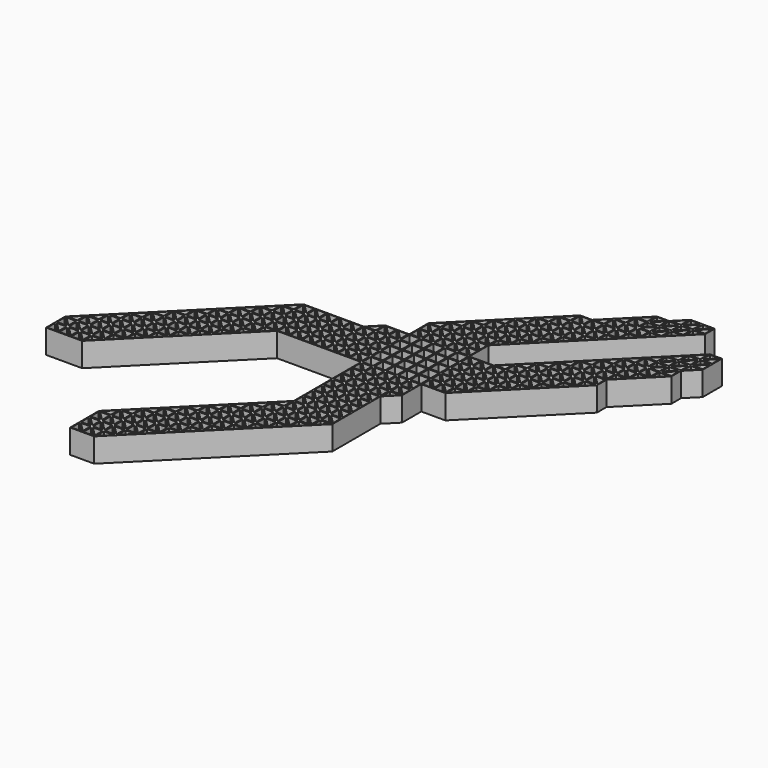
from build123d import *

# Parameters (mm, degrees)
F0_W     = 4.399904
F0_H     = 4.399732
F0_W_2   = 4.399732
F0_H_2   = 4.399903
F0_W_3   = 4.399903
F0_H_3   = 4.399904
F0_H_4   = 4.399731
F1_DEPTH = 5


with BuildPart() as f1:
    # F0 (on Top) → F1 (new body, symmetric)
    with BuildSketch(Plane.XY):
        Polygon((-42.49999, -77.500007), (-42.49999, -92.499952), (-32.500084, -92.499952), (22.500004, -37.500037), (22.500004, -12.500012), (27.500044, -7.500145), (27.500044, 2.499934), (37.500122, 2.499934), (72.500053, 37.500037), (72.500053, 42.499904), (87.499999, 57.500022), (87.499999, 62.500061), (92.500038, 67.499928), (92.500038, 77.500007), (87.499999, 77.500007), (37.49995, 27.499958), (27.500044, 27.499958), (27.500044, 37.500037), (77.500093, 87.499913), (77.500093, 92.499953), (67.500014, 92.499953), (62.499975, 87.499913), (57.500108, 87.499913), (42.49999, 72.499968), (37.500122, 72.499968), (2.500019, 37.499864), (2.500019, 27.499958), (-7.499887, 27.499958), (-12.499926, 22.499919), (-37.499951, 22.499919), (-92.500039, -32.499997), (-92.500039, -42.500076), (-77.500093, -42.500076), (-32.500084, 2.499934), (2.500019, 2.499934), (2.500019, -32.499997), align=None)
        Polygon((-42.200267, -92.199885), (-42.200267, -88.224244), (-38.224454, -92.199885), align=None, mode=Mode.SUBTRACT)
        Polygon((-37.800191, -91.775793), (-41.776003, -87.800153), (-37.800191, -87.800153), align=None, mode=Mode.SUBTRACT)
        Polygon((-37.200055, -92.199885), (-37.200055, -88.224244), (-33.224415, -92.199885), align=None, mode=Mode.SUBTRACT)
        Polygon((-36.77493, -87.800498), (-32.800496, -87.800153), (-32.800496, -91.775104), align=None, mode=Mode.SUBTRACT)
        Polygon((-42.200784, -87.200018), (-42.200784, -83.224377), (-38.224971, -87.200018), align=None, mode=Mode.SUBTRACT)
        Polygon((-41.77652, -82.800286), (-37.800708, -82.800114), (-37.800708, -86.775926), align=None, mode=Mode.SUBTRACT)
        Polygon((-37.200572, -83.224377), (-33.225104, -87.199673), (-37.200572, -87.199673), align=None, mode=Mode.SUBTRACT)
        Polygon((-32.800668, -86.775582), (-36.776308, -82.800114), (-32.800668, -82.800114), align=None, mode=Mode.SUBTRACT)
        Polygon((-28.22472, -87.800153), (-32.199844, -91.775104), (-32.199844, -87.800153), align=None, mode=Mode.SUBTRACT)
        Polygon((-28.22472, -87.200018), (-32.20036, -87.200018), (-32.20036, -83.224722), align=None, mode=Mode.SUBTRACT)
        Polygon((-27.800457, -82.800114), (-27.800457, -86.775926), (-31.776269, -82.800286), align=None, mode=Mode.SUBTRACT)
        Polygon((-23.224681, -82.800114), (-27.200321, -86.775926), (-27.200321, -82.800114), align=None, mode=Mode.SUBTRACT)
        Polygon((-42.200784, -78.22451), (-38.224971, -82.199978), (-42.200611, -82.199978), align=None, mode=Mode.SUBTRACT)
        Polygon((-37.800708, -77.800074), (-37.800708, -81.775715), (-41.77652, -77.800247), align=None, mode=Mode.SUBTRACT)
        Polygon((-37.200572, -82.199978), (-37.200572, -78.22451), (-33.22476, -82.199978), align=None, mode=Mode.SUBTRACT)
        Polygon((-32.800496, -77.800074), (-32.800496, -81.775715), (-36.776308, -77.800247), align=None, mode=Mode.SUBTRACT)
        Polygon((-41.776003, -77.199939), (-37.800535, -73.224471), (-37.800535, -77.199939), align=None, mode=Mode.SUBTRACT)
        Polygon((-37.200227, -73.224643), (-33.224587, -77.199939), (-37.200227, -77.199939), align=None, mode=Mode.SUBTRACT)
        Polygon((-32.800668, -72.800207), (-32.800668, -76.775331), (-36.776136, -72.800207), align=None, mode=Mode.SUBTRACT)
        Polygon((-32.800668, -68.224604), (-32.800496, -72.1999), (-36.776136, -72.200072), align=None, mode=Mode.SUBTRACT)
        Polygon((-32.20036, -82.199806), (-32.20036, -78.224338), (-28.224548, -82.199806), align=None, mode=Mode.SUBTRACT)
        Polygon((-27.800284, -81.775542), (-31.775925, -77.800247), (-27.800284, -77.800247), align=None, mode=Mode.SUBTRACT)
        Polygon((-32.200188, -77.199939), (-32.200188, -73.224988), (-28.225065, -77.199767), align=None, mode=Mode.SUBTRACT)
        Polygon((-27.200149, -82.199978), (-27.200149, -78.224166), (-23.224336, -82.199806), align=None, mode=Mode.SUBTRACT)
        Polygon((-26.775369, -77.800419), (-22.800417, -77.800247), (-22.800417, -81.775198), align=None, mode=Mode.SUBTRACT)
        Polygon((-23.224853, -77.199767), (-27.200321, -77.199767), (-27.200321, -73.224471), align=None, mode=Mode.SUBTRACT)
        Polygon((-27.800457, -72.800207), (-27.800457, -76.775848), (-31.776269, -72.80038), align=None, mode=Mode.SUBTRACT)
        Polygon((-28.22472, -72.200072), (-32.20036, -72.200072), (-32.20036, -68.224776), align=None, mode=Mode.SUBTRACT)
        Polygon((-27.800457, -67.800168), (-27.800457, -71.775808), (-31.776269, -67.80034), align=None, mode=Mode.SUBTRACT)
        Polygon((-22.800245, -76.775848), (-26.776058, -72.800207), (-22.800417, -72.800207), align=None, mode=Mode.SUBTRACT)
        Polygon((-27.200321, -72.200072), (-27.200321, -68.224604), (-23.224509, -72.200072), align=None, mode=Mode.SUBTRACT)
        Polygon((-22.800762, -67.800168), (-22.800762, -71.775292), (-26.776058, -67.80034), align=None, mode=Mode.SUBTRACT)
        Polygon((-18.224642, -77.800074), (-22.199937, -81.77537), (-22.199937, -77.800074), align=None, mode=Mode.SUBTRACT)
        Polygon((-18.224469, -77.199939), (-22.200109, -77.199939), (-22.200109, -73.224643), align=None, mode=Mode.SUBTRACT)
        Polygon((-17.800206, -76.775675), (-21.776018, -72.800207), (-19.99766, -72.800207), (-17.800206, -72.800035), align=None, mode=Mode.SUBTRACT)
        Polygon((-20.003172, -72.200072), (-22.200109, -72.200072), (-22.200109, -68.224776), (-18.224814, -72.1999), align=None, mode=Mode.SUBTRACT)
        Polygon((-17.80055, -71.775636), (-21.77619, -67.800168), (-17.80055, -67.800168), align=None, mode=Mode.SUBTRACT)
        Polygon((-13.22443, -72.800207), (-17.20007, -76.775848), (-17.20007, -72.800207), align=None, mode=Mode.SUBTRACT)
        Polygon((-17.20007, -72.200072), (-17.20007, -68.224604), (-13.224258, -72.200072), align=None, mode=Mode.SUBTRACT)
        Polygon((-16.775807, -67.80034), (-14.998826, -67.80034), (-12.800166, -67.800168), (-12.800166, -71.775636), align=None, mode=Mode.SUBTRACT)
        Polygon((-8.224391, -67.800168), (-12.199859, -71.775636), (-12.199859, -67.800168), align=None, mode=Mode.SUBTRACT)
        Polygon((-31.776097, -67.200032), (-27.800629, -63.224565), (-27.800629, -67.200032), align=None, mode=Mode.SUBTRACT)
        Polygon((-27.200321, -63.224737), (-23.224681, -67.200032), (-27.200321, -67.200032), align=None, mode=Mode.SUBTRACT)
        Polygon((-22.80059, -62.800129), (-22.80059, -66.775597), (-26.77623, -62.800301), align=None, mode=Mode.SUBTRACT)
        Polygon((-26.775713, -62.199993), (-22.80059, -58.22487), (-22.800417, -62.199993), align=None, mode=Mode.SUBTRACT)
        Polygon((-22.200282, -67.19986), (-22.200282, -63.224737), (-18.224814, -67.19986), align=None, mode=Mode.SUBTRACT)
        Polygon((-17.800378, -62.800129), (-17.800378, -66.775769), (-21.77619, -62.800301), align=None, mode=Mode.SUBTRACT)
        Polygon((-15.00141, -67.200205), (-17.200242, -67.200205), (-17.200242, -63.224392), (-13.22443, -67.200032), align=None, mode=Mode.SUBTRACT)
        Polygon((-16.775979, -62.800129), (-12.800339, -62.800129), (-12.800339, -66.775597), align=None, mode=Mode.SUBTRACT)
        Polygon((-22.199937, -58.225042), (-18.224642, -62.199993), (-22.199937, -62.199993), align=None, mode=Mode.SUBTRACT)
        Polygon((-17.800378, -57.800089), (-17.800378, -61.77573), (-21.77619, -57.800262), align=None, mode=Mode.SUBTRACT)
        Polygon((-17.200242, -62.199993), (-17.200242, -58.224525), (-13.22443, -62.199993), align=None, mode=Mode.SUBTRACT)
        Polygon((-12.800166, -57.800089), (-12.800166, -61.77573), (-16.775979, -57.800262), align=None, mode=Mode.SUBTRACT)
        Polygon((-8.224391, -67.200032), (-12.200031, -67.200032), (-12.200031, -63.224737), align=None, mode=Mode.SUBTRACT)
        Polygon((-7.800127, -62.800129), (-7.800127, -66.775769), (-11.77594, -62.800301), align=None, mode=Mode.SUBTRACT)
        Polygon((-3.224351, -62.800129), (-7.199991, -66.775769), (-7.199991, -62.800129), align=None, mode=Mode.SUBTRACT)
        Polygon((-12.200031, -62.199821), (-12.200031, -58.224353), (-8.224218, -62.199821), align=None, mode=Mode.SUBTRACT)
        Polygon((-7.799955, -61.775557), (-11.775595, -57.800262), (-7.799955, -57.800262), align=None, mode=Mode.SUBTRACT)
        Polygon((-7.199819, -62.199993), (-7.199819, -58.224181), (-3.224007, -62.199821), align=None, mode=Mode.SUBTRACT)
        Polygon((-6.775039, -57.800434), (-2.800088, -57.800262), (-2.800088, -61.775213), align=None, mode=Mode.SUBTRACT)
        Polygon((1.775688, -57.800089), (-2.199608, -61.775385), (-2.199608, -57.800089), align=None, mode=Mode.SUBTRACT)
        Polygon((-21.775674, -57.199954), (-17.800206, -53.224486), (-17.800206, -57.199954), align=None, mode=Mode.SUBTRACT)
        Polygon((-17.199898, -53.224658), (-13.224258, -57.199954), (-17.199898, -57.199954), align=None, mode=Mode.SUBTRACT)
        Polygon((-12.800339, -52.800222), (-12.800339, -56.775346), (-16.775807, -52.800222), align=None, mode=Mode.SUBTRACT)
        Polygon((-12.800339, -48.224619), (-12.800166, -52.199914), (-16.775807, -52.200087), align=None, mode=Mode.SUBTRACT)
        Polygon((-12.199859, -57.199954), (-12.199859, -53.225003), (-8.224735, -57.199782), align=None, mode=Mode.SUBTRACT)
        Polygon((-7.800127, -52.800222), (-7.800127, -56.775863), (-11.77594, -52.800395), align=None, mode=Mode.SUBTRACT)
        Polygon((-3.224524, -57.199782), (-7.199991, -57.199782), (-7.199991, -53.224486), align=None, mode=Mode.SUBTRACT)
        Polygon((1.77586, -57.199954), (-2.19978, -57.199954), (-2.19978, -53.224658), align=None, mode=Mode.SUBTRACT)
        Polygon((-2.799916, -56.775863), (-6.775728, -52.800222), (-2.800088, -52.800222), align=None, mode=Mode.SUBTRACT)
        Polygon((-8.224391, -52.200087), (-12.200031, -52.200087), (-12.200031, -48.224791), align=None, mode=Mode.SUBTRACT)
        Polygon((-7.800127, -47.800183), (-7.800127, -51.775823), (-11.77594, -47.800355), align=None, mode=Mode.SUBTRACT)
        Polygon((-7.199991, -52.200087), (-7.199991, -48.224619), (-3.224179, -52.200087), align=None, mode=Mode.SUBTRACT)
        Polygon((-2.800432, -47.800183), (-2.800432, -51.775306), (-6.775728, -47.800355), align=None, mode=Mode.SUBTRACT)
        Polygon((-0.002842, -52.199914), (-2.19978, -52.200087), (-2.19978, -48.224791), (1.775516, -52.199914), align=None, mode=Mode.SUBTRACT)
        Polygon((-92.200143, -42.20018), (-92.200143, -38.224368), (-88.224331, -42.20018), align=None, mode=Mode.SUBTRACT)
        Polygon((-87.800067, -41.775917), (-91.77588, -37.800104), (-87.800067, -37.800104), align=None, mode=Mode.SUBTRACT)
        Polygon((-92.199799, -37.199969), (-92.199799, -33.224156), (-88.223986, -37.199969), align=None, mode=Mode.SUBTRACT)
        Polygon((-87.800067, -32.80041), (-87.800412, -36.775016), (-91.775019, -32.80041), align=None, mode=Mode.SUBTRACT)
        Polygon((-87.199932, -42.200697), (-87.199932, -38.224885), (-83.224464, -42.200697), align=None, mode=Mode.SUBTRACT)
        Polygon((-82.8002, -41.776434), (-86.775668, -37.800621), (-82.8002, -37.800621), align=None, mode=Mode.SUBTRACT)
        Polygon((-87.199587, -37.200485), (-87.199587, -33.225018), (-83.224464, -37.200485), align=None, mode=Mode.SUBTRACT)
        Polygon((-82.8002, -36.776222), (-86.775496, -32.800582), (-82.8002, -32.800582), align=None, mode=Mode.SUBTRACT)
        Polygon((-82.200065, -42.200525), (-82.200065, -38.224885), (-78.224597, -42.200697), align=None, mode=Mode.SUBTRACT)
        Polygon((-81.775801, -37.800621), (-77.799989, -37.800621), (-77.800161, -41.776606), align=None, mode=Mode.SUBTRACT)
        Polygon((-77.199853, -41.775917), (-77.199853, -37.800449), (-73.224385, -37.800449), align=None, mode=Mode.SUBTRACT)
        Polygon((-82.200065, -37.200485), (-82.200065, -33.224673), (-78.224597, -37.200485), align=None, mode=Mode.SUBTRACT)
        Polygon((-77.799989, -32.80041), (-77.800161, -36.776394), (-81.775801, -32.80041), align=None, mode=Mode.SUBTRACT)
        Polygon((-73.224557, -37.200141), (-77.199853, -37.200141), (-77.199853, -33.224501), align=None, mode=Mode.SUBTRACT)
        Polygon((-76.775245, -32.800582), (-72.800122, -32.800582), (-72.800122, -36.77605), align=None, mode=Mode.SUBTRACT)
        Polygon((-72.199986, -36.77605), (-72.199986, -32.80041), (-68.224518, -32.800582), align=None, mode=Mode.SUBTRACT)
        Polygon((-87.800067, -28.224634), (-87.800067, -32.199757), (-91.775363, -32.199757), align=None, mode=Mode.SUBTRACT)
        Polygon((-87.199932, -28.224634), (-83.224636, -32.200274), (-87.199932, -32.200274), align=None, mode=Mode.SUBTRACT)
        Polygon((-82.8002, -27.80037), (-82.8002, -31.776183), (-86.775668, -27.80037), align=None, mode=Mode.SUBTRACT)
        Polygon((-86.775841, -27.200235), (-82.8002, -23.224594), (-82.8002, -27.200235), align=None, mode=Mode.SUBTRACT)
        Polygon((-82.19972, -32.200274), (-82.19972, -28.224461), (-78.224252, -32.200274), align=None, mode=Mode.SUBTRACT)
        Polygon((-77.800333, -27.800198), (-77.800333, -31.775666), (-81.775457, -27.800198), align=None, mode=Mode.SUBTRACT)
        Polygon((-73.225074, -32.200102), (-77.199853, -32.200102), (-77.199853, -28.224978), align=None, mode=Mode.SUBTRACT)
        Polygon((-72.800122, -27.80037), (-72.800294, -31.776355), (-76.775934, -27.80037), align=None, mode=Mode.SUBTRACT)
        Polygon((-72.199986, -32.200274), (-72.199986, -28.224634), (-68.22469, -32.200274), align=None, mode=Mode.SUBTRACT)
        Polygon((-67.800255, -27.80037), (-67.800255, -31.776183), (-71.775723, -27.80037), align=None, mode=Mode.SUBTRACT)
        Polygon((-82.199892, -23.224078), (-78.224252, -27.200062), (-82.200065, -27.200062), align=None, mode=Mode.SUBTRACT)
        Polygon((-77.800333, -22.800331), (-77.800333, -26.775454), (-81.775112, -22.800331), align=None, mode=Mode.SUBTRACT)
        Polygon((-77.199853, -27.200235), (-77.199853, -23.224767), (-73.224385, -27.200235), align=None, mode=Mode.SUBTRACT)
        Polygon((-72.800122, -26.775971), (-76.775934, -22.800159), (-72.800122, -22.800331), align=None, mode=Mode.SUBTRACT)
        Polygon((-72.199986, -27.200235), (-72.199986, -23.224422), (-68.224518, -27.200235), align=None, mode=Mode.SUBTRACT)
        Polygon((-67.800255, -26.775971), (-71.775206, -22.800675), (-67.800255, -22.800675), align=None, mode=Mode.SUBTRACT)
        Polygon((-67.200119, -31.776183), (-67.200119, -27.800542), (-63.224479, -27.800542), align=None, mode=Mode.SUBTRACT)
        Polygon((-67.200119, -27.200235), (-67.200119, -23.224594), (-63.224823, -27.200235), align=None, mode=Mode.SUBTRACT)
        Polygon((-66.775683, -22.800503), (-62.800043, -22.800503), (-62.800215, -26.776316), align=None, mode=Mode.SUBTRACT)
        Polygon((-62.199907, -26.775627), (-62.199907, -22.800331), (-58.224784, -22.800503), align=None, mode=Mode.SUBTRACT)
        Polygon((-77.799989, -18.224555), (-77.799989, -22.199851), (-81.775457, -22.199851), align=None, mode=Mode.SUBTRACT)
        Polygon((-77.199853, -22.200023), (-77.199853, -18.224383), (-73.224557, -22.200023), align=None, mode=Mode.SUBTRACT)
        Polygon((-72.800122, -17.800119), (-72.800122, -21.775932), (-76.77559, -17.800119), align=None, mode=Mode.SUBTRACT)
        Polygon((-72.199986, -18.224727), (-68.22469, -22.200023), (-72.199986, -22.200023), align=None, mode=Mode.SUBTRACT)
        Polygon((-71.775723, -17.800464), (-67.800255, -17.800464), (-67.800255, -21.775932), align=None, mode=Mode.SUBTRACT)
        Polygon((-76.775934, -17.199984), (-72.800122, -13.224343), (-72.800122, -17.199984), align=None, mode=Mode.SUBTRACT)
        Polygon((-72.199986, -17.199984), (-72.199986, -13.224171), (-68.224518, -17.199984), align=None, mode=Mode.SUBTRACT)
        Polygon((-67.800255, -12.80008), (-67.800255, -16.77572), (-71.77555, -12.80008), align=None, mode=Mode.SUBTRACT)
        Polygon((-67.800255, -8.224304), (-67.800255, -12.199772), (-71.775723, -12.199772), align=None, mode=Mode.SUBTRACT)
        Polygon((-63.224823, -22.200195), (-67.199774, -22.200195), (-67.199774, -18.2249), align=None, mode=Mode.SUBTRACT)
        Polygon((-62.800043, -17.800464), (-62.800215, -21.776276), (-66.775855, -17.800292), (-65.000081, -17.800292), align=None, mode=Mode.SUBTRACT)
        Polygon((-62.199907, -22.199851), (-62.199907, -18.224727), (-58.224956, -22.199851), align=None, mode=Mode.SUBTRACT)
        Polygon((-57.800176, -21.776104), (-61.775644, -17.800464), (-57.800176, -17.800464), align=None, mode=Mode.SUBTRACT)
        Polygon((-67.200119, -13.224343), (-63.224307, -17.200328), (-65.000081, -17.200156), (-67.200119, -17.200156), align=None, mode=Mode.SUBTRACT)
        Polygon((-62.800043, -12.800252), (-62.800043, -16.776065), (-66.775683, -12.800252), align=None, mode=Mode.SUBTRACT)
        Polygon((-62.199907, -17.200328), (-62.199907, -13.224516), (-58.224439, -17.200328), align=None, mode=Mode.SUBTRACT)
        Polygon((-57.800176, -12.800252), (-57.800176, -16.776065), (-61.775644, -12.800252), align=None, mode=Mode.SUBTRACT)
        Polygon((-53.224228, -17.800119), (-57.20004, -21.775759), (-57.20004, -17.800119), align=None, mode=Mode.SUBTRACT)
        Polygon((-57.20004, -17.199984), (-57.20004, -13.224171), (-53.224572, -17.199984), align=None, mode=Mode.SUBTRACT)
        Polygon((-56.775432, -12.800252), (-52.800309, -12.800252), (-52.800309, -16.77572), align=None, mode=Mode.SUBTRACT)
        Polygon((-48.224361, -12.800252), (-52.200173, -16.775892), (-52.199829, -12.800252), align=None, mode=Mode.SUBTRACT)
        Polygon((-67.200119, -8.224304), (-63.224651, -12.200117), (-67.200119, -12.199944), align=None, mode=Mode.SUBTRACT)
        Polygon((-62.800043, -7.800041), (-62.800215, -11.776025), (-66.775855, -7.800041), align=None, mode=Mode.SUBTRACT)
        Polygon((-62.199907, -12.200117), (-62.199907, -8.224304), (-58.224439, -12.200117), align=None, mode=Mode.SUBTRACT)
        Polygon((-57.800176, -7.800041), (-57.800176, -11.775853), (-61.775644, -7.800041), align=None, mode=Mode.SUBTRACT)
        Polygon((-66.775855, -7.199905), (-62.800043, -3.224265), (-62.800043, -7.199905), align=None, mode=Mode.SUBTRACT)
        Polygon((-62.199907, -3.224093), (-58.224095, -7.199905), (-62.199907, -7.199905), align=None, mode=Mode.SUBTRACT)
        Polygon((-57.800176, -2.800174), (-57.80052, -6.774952), (-61.775299, -2.800174), align=None, mode=Mode.SUBTRACT)
        Polygon((-57.800176, 1.775775), (-57.800176, -2.199693), (-61.775472, -2.199693), align=None, mode=Mode.SUBTRACT)
        Polygon((-53.224917, -12.199772), (-57.20004, -12.199772), (-57.199696, -8.224649), align=None, mode=Mode.SUBTRACT)
        Polygon((-52.800309, -7.800041), (-52.800309, -11.775853), (-56.775777, -7.800041), align=None, mode=Mode.SUBTRACT)
        Polygon((-48.224705, -12.200117), (-52.200173, -12.200117), (-52.200173, -8.224304), align=None, mode=Mode.SUBTRACT)
        Polygon((-47.800097, -7.800041), (-47.80027, -11.776025), (-51.77591, -7.800041), align=None, mode=Mode.SUBTRACT)
        Polygon((-57.199696, -7.199905), (-57.199696, -3.224437), (-53.224572, -7.199905), align=None, mode=Mode.SUBTRACT)
        Polygon((-52.800309, -6.775641), (-56.775777, -2.799829), (-52.800309, -2.800174), align=None, mode=Mode.SUBTRACT)
        Polygon((-57.20004, 1.775775), (-53.224917, -2.199693), (-57.20004, -2.199693), align=None, mode=Mode.SUBTRACT)
        Polygon((-52.200173, -7.199905), (-52.200173, -3.224093), (-48.224705, -7.199905), align=None, mode=Mode.SUBTRACT)
        Polygon((-47.80027, -6.775814), (-51.775221, -2.800518), (-47.800097, -2.800518), align=None, mode=Mode.SUBTRACT)
        Polygon((-52.199829, 1.77543), (-48.22505, -2.199693), (-52.200173, -2.199693), align=None, mode=Mode.SUBTRACT)
        Polygon((-11.775767, -47.200047), (-7.800299, -43.224579), (-7.800299, -47.200047), align=None, mode=Mode.SUBTRACT)
        Polygon((-7.199991, -43.224752), (-3.224351, -47.200047), (-7.199991, -47.200047), align=None, mode=Mode.SUBTRACT)
        Polygon((-2.800432, -42.800144), (-2.800432, -46.775439), (-6.7759, -42.800316), align=None, mode=Mode.SUBTRACT)
        Polygon((1.775344, -47.199875), (-2.199952, -47.199875), (-2.199952, -43.224924), align=None, mode=Mode.SUBTRACT)
        Polygon((-6.775728, -42.200008), (-2.800432, -38.224712), (-2.80026, -42.200008), align=None, mode=Mode.SUBTRACT)
        Polygon((-2.199952, -38.224885), (1.775516, -42.200008), (-2.199952, -42.200008), align=None, mode=Mode.SUBTRACT)
        Polygon((-47.199962, -11.775853), (-47.199962, -7.800385), (-43.224666, -7.800385), align=None, mode=Mode.SUBTRACT)
        Polygon((-47.199962, -7.199905), (-47.199962, -3.224437), (-43.224838, -7.199905), align=None, mode=Mode.SUBTRACT)
        Polygon((-42.80023, -6.775986), (-46.775354, -2.800518), (-42.80023, -2.800518), align=None, mode=Mode.SUBTRACT)
        Polygon((-47.199962, 1.77543), (-43.224838, -2.200038), (-47.199962, -2.200038), align=None, mode=Mode.SUBTRACT)
        Polygon((-42.200095, -6.775814), (-42.200095, -2.800174), (-38.224627, -2.800518), align=None, mode=Mode.SUBTRACT)
        Polygon((-42.200095, -2.200038), (-42.200095, 1.77543), (-38.224971, -2.200038), align=None, mode=Mode.SUBTRACT)
        Polygon((-1.775689, -52.800222), (0.00267, -52.80005), (2.199779, -52.80005), (2.199779, -56.775346), align=None, mode=Mode.SUBTRACT)
        Polygon((2.800259, -56.775346), (2.800259, -52.800222), (6.775383, -52.800222), align=None, mode=Mode.SUBTRACT)
        Polygon((-1.775861, -47.800183), (2.199779, -47.800183), (2.199779, -51.775651), align=None, mode=Mode.SUBTRACT)
        Polygon((2.800087, -52.199914), (2.799915, -48.224619), (6.775555, -52.199914), align=None, mode=Mode.SUBTRACT)
        Polygon((7.199819, -51.775651), (3.224178, -47.800355), (4.999953, -47.800183), (7.199819, -47.800183), align=None, mode=Mode.SUBTRACT)
        Polygon((11.775594, -47.800183), (7.800127, -51.775651), (7.800127, -47.800183), align=None, mode=Mode.SUBTRACT)
        Polygon((2.199779, -42.800144), (2.199779, -46.775784), (-1.776033, -42.800316), align=None, mode=Mode.SUBTRACT)
        Polygon((4.999953, -47.200047), (2.799915, -47.20022), (2.799915, -43.224407), (6.775727, -47.200047), align=None, mode=Mode.SUBTRACT)
        Polygon((7.199819, -46.775612), (3.224178, -42.800144), (7.199646, -42.800144), align=None, mode=Mode.SUBTRACT)
        Polygon((7.800127, -47.200047), (7.800127, -43.224924), (11.775594, -47.200047), align=None, mode=Mode.SUBTRACT)
        Polygon((12.199858, -42.800144), (12.199858, -46.775784), (8.224046, -42.800316), align=None, mode=Mode.SUBTRACT)
        Polygon((2.199779, -37.800104), (2.199779, -41.775745), (-1.776033, -37.800277), align=None, mode=Mode.SUBTRACT)
        Polygon((2.799915, -42.200008), (2.799915, -38.22454), (6.775727, -42.200008), align=None, mode=Mode.SUBTRACT)
        Polygon((3.224178, -37.800277), (7.199819, -37.800277), (7.199991, -41.775745), align=None, mode=Mode.SUBTRACT)
        Polygon((-1.775861, -37.199969), (2.199607, -33.224501), (2.199779, -37.199969), align=None, mode=Mode.SUBTRACT)
        Polygon((2.799915, -33.224845), (6.775383, -37.199969), (2.799915, -37.200141), align=None, mode=Mode.SUBTRACT)
        Polygon((7.199819, -32.800237), (7.199819, -36.775877), (3.224006, -32.80041), align=None, mode=Mode.SUBTRACT)
        Polygon((7.800127, -42.200008), (7.800127, -38.224712), (11.775767, -42.200008), align=None, mode=Mode.SUBTRACT)
        Polygon((12.20003, -41.775745), (8.224218, -37.800277), (12.199858, -37.800104), align=None, mode=Mode.SUBTRACT)
        Polygon((7.799954, -33.224501), (11.775767, -37.199969), (7.800127, -37.199969), align=None, mode=Mode.SUBTRACT)
        Polygon((12.20003, -36.775705), (8.224218, -32.800237), (12.199858, -32.800065), align=None, mode=Mode.SUBTRACT)
        Polygon((16.775634, -42.800144), (12.799994, -46.775784), (12.799994, -42.800144), align=None, mode=Mode.SUBTRACT)
        Polygon((12.800166, -42.200008), (12.800166, -38.224712), (16.775806, -42.200008), align=None, mode=Mode.SUBTRACT)
        Polygon((13.224257, -37.800277), (17.199897, -37.800104), (17.199897, -41.775572), align=None, mode=Mode.SUBTRACT)
        Polygon((16.775806, -37.199969), (12.800166, -37.199969), (12.800166, -33.224673), align=None, mode=Mode.SUBTRACT)
        Polygon((17.20007, -36.775705), (13.224257, -32.800237), (17.199897, -32.800065), align=None, mode=Mode.SUBTRACT)
        Polygon((21.775673, -37.800104), (17.800205, -41.775572), (17.800205, -37.800104), align=None, mode=Mode.SUBTRACT)
        Polygon((17.800205, -37.199969), (17.800205, -33.224673), (21.775845, -37.199969), align=None, mode=Mode.SUBTRACT)
        Polygon((22.200109, -36.775705), (18.224296, -32.800237), (22.200109, -32.800065), align=None, mode=Mode.SUBTRACT)
        Polygon((2.799743, -28.224461), (6.775555, -32.199929), (2.799915, -32.199929), align=None, mode=Mode.SUBTRACT)
        Polygon((3.224006, -27.800198), (7.199819, -27.800198), (7.199819, -31.775666), align=None, mode=Mode.SUBTRACT)
        Polygon((7.799954, -32.199929), (7.799954, -28.224289), (11.775767, -32.199929), align=None, mode=Mode.SUBTRACT)
        Polygon((8.22439, -27.800198), (12.199686, -27.800198), (12.199686, -30.000064), (12.199858, -31.775838), align=None, mode=Mode.SUBTRACT)
        Polygon((2.799915, -23.224594), (6.775555, -27.19989), (2.800087, -27.200062), align=None, mode=Mode.SUBTRACT)
        Polygon((3.224178, -22.800331), (4.999953, -22.800159), (7.199991, -22.800159), (7.199991, -26.775799), align=None, mode=Mode.SUBTRACT)
        Polygon((7.800127, -23.224422), (11.775594, -27.19989), (7.800127, -27.19989), align=None, mode=Mode.SUBTRACT)
        Polygon((12.199858, -22.800159), (12.20003, -25.000197), (12.20003, -26.775971), (8.224218, -22.800159), align=None, mode=Mode.SUBTRACT)
        Polygon((12.799821, -30.266886), (12.799821, -28.224289), (16.775634, -32.199929), (12.799994, -32.199929), align=None, mode=Mode.SUBTRACT)
        Polygon((13.224257, -27.800198), (17.199553, -27.800198), (17.199725, -31.775494), align=None, mode=Mode.SUBTRACT)
        Polygon((21.775501, -32.199929), (17.800033, -32.199929), (17.800033, -28.224634), align=None, mode=Mode.SUBTRACT)
        Polygon((22.199764, -31.775666), (18.224124, -27.800198), (22.199764, -27.800198), align=None, mode=Mode.SUBTRACT)
        Polygon((12.800166, -25.267019), (12.799994, -23.224422), (16.775634, -27.19989), (12.800166, -27.19989), align=None, mode=Mode.SUBTRACT)
        Polygon((17.199897, -26.775627), (13.224257, -22.800159), (17.199725, -22.800159), align=None, mode=Mode.SUBTRACT)
        Polygon((21.775501, -27.19989), (17.800205, -27.19989), (17.800205, -23.224767), align=None, mode=Mode.SUBTRACT)
        Polygon((22.199937, -26.775799), (18.224124, -22.800159), (22.199937, -22.800159), align=None, mode=Mode.SUBTRACT)
        Polygon((2.799915, -18.224383), (6.775727, -22.200023), (4.999953, -22.200023), (2.799915, -22.200195), align=None, mode=Mode.SUBTRACT)
        Polygon((7.199991, -17.800119), (7.199991, -21.775759), (3.224178, -17.800119), align=None, mode=Mode.SUBTRACT)
        Polygon((7.800127, -22.200023), (7.800127, -18.224383), (11.775594, -22.200023), align=None, mode=Mode.SUBTRACT)
        Polygon((12.199858, -17.800119), (12.199858, -21.775759), (8.22439, -17.800119), align=None, mode=Mode.SUBTRACT)
        Polygon((2.799915, -13.224516), (6.775727, -17.199984), (2.799915, -17.199984), align=None, mode=Mode.SUBTRACT)
        Polygon((3.224178, -12.800252), (7.199991, -12.800252), (7.199991, -16.77572), align=None, mode=Mode.SUBTRACT)
        Polygon((7.800127, -17.199984), (7.800127, -13.224343), (11.775594, -17.199984), align=None, mode=Mode.SUBTRACT)
        Polygon((8.224562, -12.800252), (12.199858, -12.800252), (12.199858, -16.77572), align=None, mode=Mode.SUBTRACT)
        Polygon((12.799994, -22.200023), (12.799994, -18.224383), (16.775806, -22.200023), align=None, mode=Mode.SUBTRACT)
        Polygon((17.199725, -21.775415), (13.224257, -17.800119), (17.199725, -17.800119), align=None, mode=Mode.SUBTRACT)
        Polygon((17.800205, -22.200023), (17.800205, -18.224727), (21.775673, -22.200023), align=None, mode=Mode.SUBTRACT)
        Polygon((22.199937, -21.775759), (18.224124, -17.800119), (22.199937, -17.800119), align=None, mode=Mode.SUBTRACT)
        Polygon((12.799994, -17.199984), (12.799994, -13.224343), (16.775806, -17.199984), align=None, mode=Mode.SUBTRACT)
        Polygon((17.199725, -16.775376), (13.224429, -12.800252), (17.199725, -12.800252), align=None, mode=Mode.SUBTRACT)
        Polygon((17.800205, -17.199984), (17.800205, -13.224688), (21.775673, -17.199984), align=None, mode=Mode.SUBTRACT)
        Polygon((22.199937, -16.77572), (18.224296, -12.800252), (22.199937, -12.800252), align=None, mode=Mode.SUBTRACT)
        Polygon((2.799743, -8.224649), (6.775383, -12.199944), (2.799915, -12.200117), align=None, mode=Mode.SUBTRACT)
        Polygon((3.224006, -7.800385), (4.999781, -7.800213), (7.199819, -7.800213), (7.199819, -11.775853), align=None, mode=Mode.SUBTRACT)
        Polygon((7.799954, -8.224476), (11.775594, -12.199944), (7.799954, -12.199944), align=None, mode=Mode.SUBTRACT)
        Polygon((12.199686, -7.800213), (12.199686, -10.000251), (12.199858, -11.776025), (8.224218, -7.800213), align=None, mode=Mode.SUBTRACT)
        Polygon((2.799743, -3.224437), (6.775555, -7.200077), (4.999781, -7.200077), (2.799743, -7.200249), align=None, mode=Mode.SUBTRACT)
        Polygon((7.199819, -2.800174), (7.199819, -6.775814), (3.224006, -2.800174), align=None, mode=Mode.SUBTRACT)
        Polygon((2.799743, 1.77543), (6.775555, -2.200038), (2.799743, -2.200038), align=None, mode=Mode.SUBTRACT)
        Polygon((7.799954, -7.200077), (7.799954, -3.224437), (11.775422, -7.200077), align=None, mode=Mode.SUBTRACT)
        Polygon((12.199686, -2.800174), (12.199686, -6.775814), (8.224218, -2.800174), align=None, mode=Mode.SUBTRACT)
        Polygon((7.799954, -2.200038), (7.799954, 1.775602), (11.775422, -2.200038), align=None, mode=Mode.SUBTRACT)
        Polygon((12.799821, -10.267073), (12.799821, -8.224476), (16.775462, -12.199944), (12.799994, -12.199944), align=None, mode=Mode.SUBTRACT)
        Polygon((17.199553, -7.800213), (17.199725, -11.775681), (13.224085, -7.800213), align=None, mode=Mode.SUBTRACT)
        Polygon((17.800033, -12.199944), (17.800033, -8.224821), (21.775329, -12.199944), align=None, mode=Mode.SUBTRACT)
        Polygon((22.199592, -11.775681), (18.223952, -7.800213), (22.199592, -7.800213), align=None, mode=Mode.SUBTRACT)
        Polygon((12.799821, -7.200077), (12.799821, -3.224437), (16.775634, -7.200077), align=None, mode=Mode.SUBTRACT)
        Polygon((13.224085, -2.800174), (17.199553, -2.800174), (17.199553, -6.775469), align=None, mode=Mode.SUBTRACT)
        Polygon((12.799821, -2.200038), (12.799821, 1.775602), (16.775634, -2.200038), align=None, mode=Mode.SUBTRACT)
        Polygon((21.775501, -7.200077), (17.800033, -7.200077), (17.800033, -3.224782), align=None, mode=Mode.SUBTRACT)
        Polygon((22.199764, -2.800174), (22.199764, -6.775814), (18.223952, -2.800174), align=None, mode=Mode.SUBTRACT)
        Polygon((17.800033, -2.200038), (17.800033, 1.775258), (21.775501, -2.200038), align=None, mode=Mode.SUBTRACT)
        Polygon((26.775368, -7.800213), (22.7999, -11.775681), (22.7999, -7.800213), align=None, mode=Mode.SUBTRACT)
        Polygon((22.7999, -7.200077), (22.7999, -3.224437), (26.775368, -7.200077), align=None, mode=Mode.SUBTRACT)
        Polygon((27.199631, -2.800174), (27.199631, -6.775814), (23.224164, -2.800174), align=None, mode=Mode.SUBTRACT)
        Polygon((26.775368, -2.200038), (22.7999, -2.200038), (22.7999, 1.775602), align=None, mode=Mode.SUBTRACT)
        Polygon((-52.799964, 2.199694), (-52.800309, -1.775774), (-56.775432, 2.199694), align=None, mode=Mode.SUBTRACT)
        Polygon((-52.800309, 6.775297), (-52.800309, 2.800174), (-56.775432, 2.800174), align=None, mode=Mode.SUBTRACT)
        Polygon((-47.800097, 2.199694), (-47.800097, -1.776119), (-51.775565, 2.199694), align=None, mode=Mode.SUBTRACT)
        Polygon((-48.224705, 2.799829), (-52.199829, 2.800001), (-52.199829, 6.775297), align=None, mode=Mode.SUBTRACT)
        Polygon((-47.800097, 7.199905), (-47.800442, 3.224093), (-51.77591, 7.199905), align=None, mode=Mode.SUBTRACT)
        Polygon((-51.77591, 7.800041), (-47.800097, 11.775681), (-47.800097, 7.800041), align=None, mode=Mode.SUBTRACT)
        Polygon((-42.80023, 2.199694), (-42.80023, -1.776119), (-46.775698, 2.199694), align=None, mode=Mode.SUBTRACT)
        Polygon((-43.224494, 2.799829), (-47.200306, 2.799829), (-47.199962, 6.775642), align=None, mode=Mode.SUBTRACT)
        Polygon((-42.80023, 3.224093), (-46.775698, 7.199905), (-42.80023, 7.199561), align=None, mode=Mode.SUBTRACT)
        Polygon((-37.800019, 2.199694), (-37.800191, -1.776291), (-41.775831, 2.199694), align=None, mode=Mode.SUBTRACT)
        Polygon((-33.224415, 2.199694), (-37.199883, -1.775774), (-37.199883, 2.199694), align=None, mode=Mode.SUBTRACT)
        Polygon((-42.200095, 2.799829), (-42.200095, 6.775642), (-38.224627, 2.799829), align=None, mode=Mode.SUBTRACT)
        Polygon((-37.800363, 3.224093), (-41.775831, 7.199905), (-37.800363, 7.199905), align=None, mode=Mode.SUBTRACT)
        Polygon((-33.22476, 2.799829), (-37.200227, 2.799829), (-37.199883, 6.775297), align=None, mode=Mode.SUBTRACT)
        Polygon((-32.800152, 7.199905), (-32.800324, 3.22392), (-36.775964, 7.199905), align=None, mode=Mode.SUBTRACT)
        Polygon((-47.199962, 11.775509), (-43.224838, 7.800041), (-47.199962, 7.800041), align=None, mode=Mode.SUBTRACT)
        Polygon((-42.80023, 12.199772), (-42.80023, 8.22396), (-46.775698, 12.199772), align=None, mode=Mode.SUBTRACT)
        Polygon((-42.200095, 7.800041), (-42.200095, 11.775853), (-38.224627, 7.800041), align=None, mode=Mode.SUBTRACT)
        Polygon((-41.775831, 12.200117), (-37.800019, 12.199772), (-37.800191, 8.224132), align=None, mode=Mode.SUBTRACT)
        Polygon((-37.199883, 7.800041), (-37.199883, 11.775853), (-33.224415, 7.800041), align=None, mode=Mode.SUBTRACT)
        Polygon((-32.800152, 8.224304), (-36.775619, 12.200117), (-32.800152, 12.199772), align=None, mode=Mode.SUBTRACT)
        Polygon((-32.200016, 2.799829), (-32.200016, 6.775642), (-28.224548, 2.799829), align=None, mode=Mode.SUBTRACT)
        Polygon((-31.775752, 7.199905), (-27.800284, 7.199905), (-27.800284, 3.224093), align=None, mode=Mode.SUBTRACT)
        Polygon((-27.200149, 2.800001), (-27.199804, 6.775297), (-23.224681, 2.799829), align=None, mode=Mode.SUBTRACT)
        Polygon((-26.775885, 7.199905), (-22.800073, 7.199905), (-22.800417, 3.224093), align=None, mode=Mode.SUBTRACT)
        Polygon((-32.200016, 7.800041), (-32.200016, 11.775509), (-28.224203, 7.800041), align=None, mode=Mode.SUBTRACT)
        Polygon((-31.775752, 12.199772), (-27.800284, 12.199772), (-27.800284, 8.224649), align=None, mode=Mode.SUBTRACT)
        Polygon((-27.199804, 7.800041), (-27.199804, 11.775509), (-23.224336, 7.800041), align=None, mode=Mode.SUBTRACT)
        Polygon((-22.800073, 8.224304), (-26.775885, 12.200117), (-22.800073, 12.199772), align=None, mode=Mode.SUBTRACT)
        Polygon((-46.77587, 12.799908), (-42.80023, 16.77572), (-42.80023, 12.799908), align=None, mode=Mode.SUBTRACT)
        Polygon((-42.200095, 16.77572), (-38.224971, 12.800252), (-42.200095, 12.800252), align=None, mode=Mode.SUBTRACT)
        Polygon((-37.800019, 17.199984), (-37.800191, 13.223999), (-41.775831, 17.199984), align=None, mode=Mode.SUBTRACT)
        Polygon((-37.199883, 16.77572), (-33.22476, 12.800252), (-37.199883, 12.800252), align=None, mode=Mode.SUBTRACT)
        Polygon((-32.800152, 17.199984), (-32.800152, 13.224171), (-36.775619, 17.199984), align=None, mode=Mode.SUBTRACT)
        Polygon((-41.775831, 17.800119), (-37.800019, 21.77576), (-37.800019, 17.800119), align=None, mode=Mode.SUBTRACT)
        Polygon((-37.199883, 21.775932), (-33.224415, 17.800119), (-37.199883, 17.800119), align=None, mode=Mode.SUBTRACT)
        Polygon((-32.800152, 22.200195), (-32.800152, 18.224383), (-36.775619, 22.200195), align=None, mode=Mode.SUBTRACT)
        Polygon((-32.200016, 12.799908), (-32.200016, 16.77572), (-28.224203, 12.799908), align=None, mode=Mode.SUBTRACT)
        Polygon((-27.800284, 17.199639), (-27.800284, 13.224516), (-31.775408, 17.199639), align=None, mode=Mode.SUBTRACT)
        Polygon((-27.199804, 12.800252), (-27.199804, 16.775376), (-23.224336, 12.799908), align=None, mode=Mode.SUBTRACT)
        Polygon((-22.800073, 13.224171), (-26.775885, 17.199984), (-22.800073, 17.199639), align=None, mode=Mode.SUBTRACT)
        Polygon((-32.200016, 21.775587), (-28.224548, 17.800119), (-32.200016, 17.800119), align=None, mode=Mode.SUBTRACT)
        Polygon((-27.800284, 22.199851), (-27.800284, 18.224383), (-31.775752, 22.199851), align=None, mode=Mode.SUBTRACT)
        Polygon((-23.224681, 17.800119), (-27.199804, 17.800119), (-27.199804, 21.775243), align=None, mode=Mode.SUBTRACT)
        Polygon((-22.800073, 22.199851), (-22.800073, 18.224038), (-26.775885, 22.199851), align=None, mode=Mode.SUBTRACT)
        Polygon((-22.200282, 2.799829), (-22.199937, 6.775642), (-18.224469, 2.799829), align=None, mode=Mode.SUBTRACT)
        Polygon((-17.800206, 3.224093), (-21.775674, 7.199905), (-17.800206, 7.199905), align=None, mode=Mode.SUBTRACT)
        Polygon((-17.20007, 2.799829), (-17.20007, 6.775642), (-13.224602, 2.799829), align=None, mode=Mode.SUBTRACT)
        Polygon((-16.775807, 7.199905), (-12.800339, 7.199905), (-12.800339, 3.224093), align=None, mode=Mode.SUBTRACT)
        Polygon((-22.199937, 7.800041), (-22.199937, 11.775681), (-18.224297, 7.800041), align=None, mode=Mode.SUBTRACT)
        Polygon((-17.800206, 12.199772), (-17.800206, 8.224132), (-21.775846, 12.199772), align=None, mode=Mode.SUBTRACT)
        Polygon((-17.20007, 7.800041), (-17.20007, 11.775509), (-13.224258, 7.800041), align=None, mode=Mode.SUBTRACT)
        Polygon((-16.775807, 12.199772), (-12.800339, 12.199772), (-12.800339, 8.224649), align=None, mode=Mode.SUBTRACT)
        Polygon((-12.200203, 2.799829), (-12.199859, 6.775297), (-8.224735, 2.799829), align=None, mode=Mode.SUBTRACT)
        Polygon((-11.77594, 7.199905), (-7.800127, 7.199905), (-7.800472, 3.224093), align=None, mode=Mode.SUBTRACT)
        Polygon((-7.200336, 2.799829), (-7.199991, 6.775642), (-3.224524, 2.799829), align=None, mode=Mode.SUBTRACT)
        Polygon((-2.80026, 3.224093), (-6.775728, 7.199905), (-2.80026, 7.199905), align=None, mode=Mode.SUBTRACT)
        Polygon((-2.200124, 2.799829), (-2.200124, 6.775642), (1.775344, 2.799829), align=None, mode=Mode.SUBTRACT)
        Polygon((-12.199859, 7.800041), (-12.199859, 11.775164), (-8.224391, 7.800041), align=None, mode=Mode.SUBTRACT)
        Polygon((-7.800127, 12.199772), (-7.800127, 8.224304), (-11.77594, 12.199772), align=None, mode=Mode.SUBTRACT)
        Polygon((-7.199991, 7.800041), (-7.199991, 11.775681), (-3.224351, 7.800041), align=None, mode=Mode.SUBTRACT)
        Polygon((-2.80026, 12.199772), (-2.80026, 8.224132), (-6.7759, 12.199772), align=None, mode=Mode.SUBTRACT)
        Polygon((-2.200124, 7.800041), (-2.200124, 11.775509), (1.775688, 7.800041), align=None, mode=Mode.SUBTRACT)
        Polygon((-22.199937, 12.799908), (-22.199937, 16.77572), (-18.224469, 12.799908), align=None, mode=Mode.SUBTRACT)
        Polygon((-17.800206, 13.224171), (-21.775329, 17.199639), (-17.800206, 17.199639), align=None, mode=Mode.SUBTRACT)
        Polygon((-17.20007, 12.799908), (-17.20007, 16.77572), (-13.224258, 12.799908), align=None, mode=Mode.SUBTRACT)
        Polygon((-12.800339, 17.199639), (-12.800339, 13.224516), (-16.775462, 17.199639), align=None, mode=Mode.SUBTRACT)
        Polygon((-22.199937, 21.775587), (-18.224814, 17.800119), (-22.199937, 17.800119), align=None, mode=Mode.SUBTRACT)
        Polygon((-17.800206, 22.199851), (-17.800206, 18.224038), (-21.775674, 22.199851), align=None, mode=Mode.SUBTRACT)
        Polygon((-17.20007, 21.775587), (-13.224602, 17.800119), (-17.20007, 17.800119), align=None, mode=Mode.SUBTRACT)
        Polygon((-12.800339, 22.199851), (-12.800339, 18.224383), (-16.775807, 22.199851), align=None, mode=Mode.SUBTRACT)
        Polygon((-12.199859, 12.799908), (-12.199859, 16.775376), (-8.224391, 12.799908), align=None, mode=Mode.SUBTRACT)
        Polygon((-7.800127, 13.224171), (-11.775595, 17.199639), (-7.800127, 17.199639), align=None, mode=Mode.SUBTRACT)
        Polygon((-7.199991, 12.799908), (-7.199991, 16.77572), (-3.224524, 12.799908), align=None, mode=Mode.SUBTRACT)
        Polygon((-2.80026, 13.224171), (-6.775383, 17.199639), (-2.80026, 17.199639), align=None, mode=Mode.SUBTRACT)
        Polygon((-2.200124, 12.799908), (-2.200124, 16.77572), (1.775688, 12.799908), align=None, mode=Mode.SUBTRACT)
        Polygon((-8.224735, 17.800119), (-12.199859, 17.800119), (-12.199859, 21.775243), align=None, mode=Mode.SUBTRACT)
        Polygon((-7.800127, 22.199506), (-7.800127, 18.224038), (-11.775595, 22.199506), align=None, mode=Mode.SUBTRACT)
        Polygon((-7.199991, 21.775587), (-3.224868, 17.800119), (-7.199991, 17.800119), align=None, mode=Mode.SUBTRACT)
        Polygon((-2.800088, 22.199851), (-2.80026, 19.999813), (-2.80026, 18.224038), (-6.775728, 22.199851), align=None, mode=Mode.SUBTRACT)
        Polygon((1.775344, 17.800119), (-2.200124, 17.800119), (-2.200124, 19.999813), (-2.199952, 21.775587), align=None, mode=Mode.SUBTRACT)
        Polygon((-7.800127, 26.775454), (-7.800127, 22.799987), (-11.775595, 22.799987), align=None, mode=Mode.SUBTRACT)
        Polygon((-7.199991, 26.775454), (-3.224351, 22.799987), (-7.199991, 22.799987), align=None, mode=Mode.SUBTRACT)
        Polygon((-2.800088, 27.199718), (-2.800088, 23.22425), (-6.775728, 27.199718), align=None, mode=Mode.SUBTRACT)
        Polygon((-2.199952, 26.775454), (1.775688, 22.799987), (-2.199952, 22.799987), align=None, mode=Mode.SUBTRACT)
        Polygon((3.224006, 2.199694), (7.199819, 2.199694), (7.199819, -1.775774), align=None, mode=Mode.SUBTRACT)
        Polygon((-1.775861, 7.199905), (2.199779, 7.199905), (2.199779, 3.22392), align=None, mode=Mode.SUBTRACT)
        Polygon((2.799915, 4.999867), (2.800087, 7.199733), (7.199819, 7.199733), (7.199819, 2.800001), (2.799915, 2.799829), align=None, mode=Mode.SUBTRACT)
        Polygon((8.22439, 2.199694), (12.199686, 2.199694), (12.199686, -1.775774), align=None, mode=Mode.SUBTRACT)
        with Locations((9.999906, 4.999867)):
            Rectangle(F0_W, F0_H, mode=Mode.SUBTRACT)
        Polygon((-1.775861, 12.199772), (2.199779, 12.199772), (2.199779, 8.224477), align=None, mode=Mode.SUBTRACT)
        with Locations((4.999953, 9.9998205)):
            Rectangle(F0_W_2, F0_H_2, mode=Mode.SUBTRACT)
        with Locations((9.999906, 9.9998205)):
            Rectangle(F0_W, F0_H_2, mode=Mode.SUBTRACT)
        Polygon((13.224257, 2.199694), (17.199553, 2.199694), (17.199553, -1.77543), align=None, mode=Mode.SUBTRACT)
        with Locations((14.9999455, 4.999867)):
            Rectangle(F0_W_3, F0_H, mode=Mode.SUBTRACT)
        Polygon((22.199764, -1.775774), (18.224124, 2.199694), (22.199764, 2.199694), align=None, mode=Mode.SUBTRACT)
        with Locations((19.999985, 4.999867)):
            Rectangle(F0_W, F0_H, mode=Mode.SUBTRACT)
        with Locations((14.9999455, 9.9998205)):
            Rectangle(F0_W_3, F0_H_2, mode=Mode.SUBTRACT)
        with Locations((19.999985, 9.9998205)):
            Rectangle(F0_W, F0_H_2, mode=Mode.SUBTRACT)
        Polygon((-1.775516, 17.199639), (2.199779, 17.199639), (2.199779, 13.224344), align=None, mode=Mode.SUBTRACT)
        with Locations((4.999953, 14.99986)):
            Rectangle(F0_W_2, F0_H_3, mode=Mode.SUBTRACT)
        with Locations((9.999906, 14.99986)):
            Rectangle(F0_W, F0_H_3, mode=Mode.SUBTRACT)
        Polygon((2.199779, 22.199851), (2.199779, 18.224211), (-1.775689, 22.199851), align=None, mode=Mode.SUBTRACT)
        with Locations((4.999953, 19.999899)):
            Rectangle(F0_W_2, F0_H_3, mode=Mode.SUBTRACT)
        with Locations((9.999906, 19.999899)):
            Rectangle(F0_W, F0_H_3, mode=Mode.SUBTRACT)
        with Locations((14.9999455, 14.99986)):
            Rectangle(F0_W_3, F0_H_3, mode=Mode.SUBTRACT)
        with Locations((19.999985, 14.99986)):
            Rectangle(F0_W, F0_H_3, mode=Mode.SUBTRACT)
        with Locations((14.9999455, 19.999899)):
            Rectangle(F0_W_3, F0_H_3, mode=Mode.SUBTRACT)
        with Locations((19.999985, 19.999899)):
            Rectangle(F0_W, F0_H_3, mode=Mode.SUBTRACT)
        Polygon((27.199631, -1.775774), (23.224336, 2.199694), (27.199631, 2.199694), align=None, mode=Mode.SUBTRACT)
        with Locations((24.999938, 4.999867)):
            Rectangle(F0_W_2, F0_H, mode=Mode.SUBTRACT)
        Polygon((27.800112, 2.800001), (27.800112, 6.775469), (31.775407, 2.799829), align=None, mode=Mode.SUBTRACT)
        Polygon((32.199671, 3.224093), (28.224203, 7.199905), (32.199843, 7.199905), (32.199843, 4.999867), align=None, mode=Mode.SUBTRACT)
        with Locations((24.999938, 9.9998205)):
            Rectangle(F0_W_2, F0_H_2, mode=Mode.SUBTRACT)
        Polygon((27.800112, 7.800041), (27.800112, 11.775509), (31.77558, 7.800041), align=None, mode=Mode.SUBTRACT)
        Polygon((32.199843, 12.199772), (32.199843, 8.224132), (28.224031, 12.199944), (29.999805, 12.199944), align=None, mode=Mode.SUBTRACT)
        Polygon((32.799806, 2.799829), (32.799979, 4.999867), (32.799979, 6.775642), (36.775619, 2.799829), align=None, mode=Mode.SUBTRACT)
        Polygon((37.199882, 3.224093), (33.224242, 7.199905), (37.199882, 7.199905), align=None, mode=Mode.SUBTRACT)
        Polygon((41.77583, 7.199905), (37.800018, 3.224093), (37.800018, 7.199905), align=None, mode=Mode.SUBTRACT)
        Polygon((32.799979, 7.800041), (32.799979, 11.775509), (36.775619, 7.800041), align=None, mode=Mode.SUBTRACT)
        Polygon((37.199882, 12.199772), (37.199882, 8.224304), (33.224242, 12.199772), align=None, mode=Mode.SUBTRACT)
        Polygon((37.800018, 7.800041), (37.800018, 11.775509), (41.775658, 7.800041), align=None, mode=Mode.SUBTRACT)
        Polygon((42.199922, 8.224304), (38.224282, 12.199772), (42.199922, 12.199772), align=None, mode=Mode.SUBTRACT)
        Polygon((46.77587, 12.199944), (42.800057, 8.224132), (42.800057, 12.199944), align=None, mode=Mode.SUBTRACT)
        with Locations((24.999938, 14.99986)):
            Rectangle(F0_W_2, F0_H_3, mode=Mode.SUBTRACT)
        Polygon((29.999805, 12.80008), (27.800112, 12.80008), (27.800112, 16.775548), (31.77558, 12.799908), align=None, mode=Mode.SUBTRACT)
        Polygon((32.199843, 13.224171), (28.224375, 17.199812), (32.199843, 17.199639), align=None, mode=Mode.SUBTRACT)
        with Locations((24.999938, 19.999899)):
            Rectangle(F0_W_2, F0_H_3, mode=Mode.SUBTRACT)
        Polygon((31.775235, 17.800119), (27.800112, 17.800119), (27.800112, 21.775415), align=None, mode=Mode.SUBTRACT)
        Polygon((32.199843, 22.199851), (32.199843, 18.224038), (28.224203, 22.199851), align=None, mode=Mode.SUBTRACT)
        Polygon((32.799979, 12.799908), (32.799979, 16.77572), (36.775619, 12.799908), align=None, mode=Mode.SUBTRACT)
        Polygon((37.199882, 13.224171), (33.224587, 17.199639), (37.199882, 17.199639), align=None, mode=Mode.SUBTRACT)
        Polygon((37.800018, 12.799908), (37.800018, 16.77572), (41.775658, 12.799908), align=None, mode=Mode.SUBTRACT)
        Polygon((38.224626, 17.199639), (42.199922, 17.199639), (42.199749, 13.224344), align=None, mode=Mode.SUBTRACT)
        Polygon((42.800057, 12.80008), (42.800057, 16.775893), (46.775698, 12.80008), align=None, mode=Mode.SUBTRACT)
        Polygon((47.199961, 17.200156), (47.199961, 13.224344), (43.224321, 17.200156), align=None, mode=Mode.SUBTRACT)
        Polygon((32.799979, 21.775587), (36.775274, 17.800119), (32.799979, 17.800119), align=None, mode=Mode.SUBTRACT)
        Polygon((37.199882, 22.199851), (37.199882, 18.224038), (33.224242, 22.199851), align=None, mode=Mode.SUBTRACT)
        Polygon((37.800018, 21.775587), (41.775314, 17.800119), (37.800018, 17.800119), align=None, mode=Mode.SUBTRACT)
        Polygon((42.199922, 22.199851), (42.199922, 18.224038), (38.224282, 22.199851), align=None, mode=Mode.SUBTRACT)
        Polygon((42.800057, 17.800292), (42.800057, 21.77576), (46.775698, 17.800292), align=None, mode=Mode.SUBTRACT)
        Polygon((47.199961, 22.200023), (47.199961, 18.224555), (43.224321, 22.200023), align=None, mode=Mode.SUBTRACT)
        Polygon((2.199779, 27.199718), (2.199779, 23.224422), (-1.775689, 27.199718), align=None, mode=Mode.SUBTRACT)
        with Locations((4.999953, 24.9998525)):
            Rectangle(F0_W_2, F0_H_4, mode=Mode.SUBTRACT)
        with Locations((9.999906, 24.9998525)):
            Rectangle(F0_W, F0_H_4, mode=Mode.SUBTRACT)
        Polygon((2.799743, 31.775322), (6.775383, 27.800026), (2.799915, 27.800026), align=None, mode=Mode.SUBTRACT)
        Polygon((3.224006, 32.199585), (4.999781, 32.199757), (7.199819, 32.199757), (7.199819, 28.224117), align=None, mode=Mode.SUBTRACT)
        Polygon((7.799954, 31.775494), (11.775594, 27.800026), (7.799954, 27.800026), align=None, mode=Mode.SUBTRACT)
        Polygon((12.199686, 32.199757), (12.199686, 29.999719), (12.199858, 28.223945), (8.224218, 32.199757), align=None, mode=Mode.SUBTRACT)
        with Locations((14.9999455, 24.9998525)):
            Rectangle(F0_W_3, F0_H_4, mode=Mode.SUBTRACT)
        with Locations((19.999985, 24.9998525)):
            Rectangle(F0_W, F0_H_4, mode=Mode.SUBTRACT)
        Polygon((12.799821, 29.732897), (12.799821, 31.775494), (16.775462, 27.800026), (12.799994, 27.800026), align=None, mode=Mode.SUBTRACT)
        Polygon((17.199553, 32.199757), (17.199725, 28.224289), (13.224085, 32.199757), align=None, mode=Mode.SUBTRACT)
        Polygon((21.775329, 27.800026), (17.800033, 27.800026), (17.800033, 31.775149), align=None, mode=Mode.SUBTRACT)
        Polygon((22.199764, 32.199757), (22.199764, 28.224117), (18.223952, 32.199757), align=None, mode=Mode.SUBTRACT)
        Polygon((2.799743, 36.775533), (6.775555, 32.799893), (4.999781, 32.799893), (2.799743, 32.799721), align=None, mode=Mode.SUBTRACT)
        Polygon((7.199819, 37.199797), (7.199819, 33.224156), (3.224006, 37.199797), align=None, mode=Mode.SUBTRACT)
        Polygon((3.224006, 37.799932), (7.199819, 41.775745), (7.199819, 37.799932), align=None, mode=Mode.SUBTRACT)
        Polygon((7.799954, 32.799893), (7.799954, 36.775533), (11.775422, 32.799893), align=None, mode=Mode.SUBTRACT)
        Polygon((12.199686, 37.199797), (12.199686, 33.224156), (8.224218, 37.199797), align=None, mode=Mode.SUBTRACT)
        Polygon((7.799954, 41.775572), (11.775422, 37.799932), (7.799954, 37.799932), align=None, mode=Mode.SUBTRACT)
        Polygon((12.199686, 42.199836), (12.199686, 38.224196), (8.224218, 42.199836), align=None, mode=Mode.SUBTRACT)
        Polygon((8.224046, 42.799972), (12.199858, 46.775784), (12.199858, 42.799972), align=None, mode=Mode.SUBTRACT)
        Polygon((12.799821, 32.799893), (12.799821, 36.775533), (16.775634, 32.799893), align=None, mode=Mode.SUBTRACT)
        Polygon((17.199553, 37.199797), (17.199553, 33.224501), (13.224085, 37.199797), align=None, mode=Mode.SUBTRACT)
        Polygon((12.799821, 37.799932), (12.799821, 41.775572), (16.775634, 37.799932), align=None, mode=Mode.SUBTRACT)
        Polygon((13.224257, 42.199664), (17.199553, 42.199836), (17.199553, 38.22454), align=None, mode=Mode.SUBTRACT)
        Polygon((17.800033, 32.799893), (17.800033, 36.775189), (21.775501, 32.799893), align=None, mode=Mode.SUBTRACT)
        Polygon((22.199764, 37.199797), (22.199764, 33.224156), (18.223952, 37.199797), align=None, mode=Mode.SUBTRACT)
        Polygon((17.800033, 37.799932), (17.800033, 41.775228), (21.775501, 37.799932), align=None, mode=Mode.SUBTRACT)
        Polygon((22.199764, 42.199836), (22.199764, 38.224196), (18.223952, 42.199836), align=None, mode=Mode.SUBTRACT)
        Polygon((12.799994, 46.775612), (16.775806, 42.799972), (12.799994, 42.799972), align=None, mode=Mode.SUBTRACT)
        Polygon((17.20007, 47.199875), (17.20007, 43.224235), (13.224257, 47.199875), align=None, mode=Mode.SUBTRACT)
        Polygon((17.800205, 42.799972), (17.800205, 46.775612), (21.775673, 42.799972), align=None, mode=Mode.SUBTRACT)
        Polygon((22.199937, 47.199875), (22.199937, 43.224235), (18.224469, 47.199875), align=None, mode=Mode.SUBTRACT)
        with Locations((24.999938, 24.9998525)):
            Rectangle(F0_W_2, F0_H_4, mode=Mode.SUBTRACT)
        Polygon((31.77558, 22.799987), (27.800112, 22.799987), (27.800112, 26.775454), align=None, mode=Mode.SUBTRACT)
        Polygon((32.199843, 27.199718), (32.199843, 23.224078), (28.224031, 27.19989), align=None, mode=Mode.SUBTRACT)
        Polygon((26.77554, 27.800026), (22.7999, 27.800026), (22.7999, 31.775494), align=None, mode=Mode.SUBTRACT)
        Polygon((27.199804, 28.223945), (23.224164, 32.199757), (27.199631, 32.199757), align=None, mode=Mode.SUBTRACT)
        Polygon((32.799979, 26.775454), (36.775619, 22.799987), (32.799979, 22.799987), align=None, mode=Mode.SUBTRACT)
        Polygon((37.199882, 27.199718), (37.199882, 23.22425), (33.224242, 27.199718), align=None, mode=Mode.SUBTRACT)
        Polygon((37.800018, 22.799987), (37.800018, 26.775454), (41.775658, 22.799987), align=None, mode=Mode.SUBTRACT)
        Polygon((42.199922, 27.199718), (42.199922, 23.22425), (38.224282, 27.199718), align=None, mode=Mode.SUBTRACT)
        Polygon((42.800057, 22.800159), (42.800057, 26.775627), (46.775698, 22.800159), align=None, mode=Mode.SUBTRACT)
        Polygon((47.199961, 27.19989), (47.199961, 23.224422), (43.224321, 27.19989), align=None, mode=Mode.SUBTRACT)
        Polygon((38.224282, 27.800026), (42.199922, 31.775666), (42.199922, 27.800026), align=None, mode=Mode.SUBTRACT)
        Polygon((42.800057, 31.775666), (46.775698, 27.800198), (42.800057, 27.800198), align=None, mode=Mode.SUBTRACT)
        Polygon((47.199961, 32.19993), (47.199961, 28.224462), (43.224321, 32.19993), align=None, mode=Mode.SUBTRACT)
        Polygon((22.7999, 32.799893), (22.7999, 36.775533), (26.775368, 32.799893), align=None, mode=Mode.SUBTRACT)
        Polygon((27.199631, 33.224156), (23.224164, 37.199797), (27.199631, 37.199797), align=None, mode=Mode.SUBTRACT)
        Polygon((22.7999, 37.799932), (22.7999, 41.775572), (26.775368, 37.799932), align=None, mode=Mode.SUBTRACT)
        Polygon((27.199631, 42.199836), (27.199631, 38.224196), (23.224164, 42.199836), align=None, mode=Mode.SUBTRACT)
        Polygon((31.77558, 42.199836), (27.799939, 38.224196), (27.799939, 42.199836), align=None, mode=Mode.SUBTRACT)
        Polygon((22.800072, 42.799972), (22.800072, 46.775612), (26.77554, 42.799972), align=None, mode=Mode.SUBTRACT)
        Polygon((27.199804, 47.199875), (27.199804, 43.224235), (23.224336, 47.199875), align=None, mode=Mode.SUBTRACT)
        Polygon((27.800112, 42.799972), (27.800112, 46.775612), (31.77558, 42.799972), align=None, mode=Mode.SUBTRACT)
        Polygon((32.199843, 47.199875), (32.199843, 43.224235), (28.224375, 47.199875), align=None, mode=Mode.SUBTRACT)
        Polygon((43.224321, 32.800065), (47.199961, 36.775705), (47.199961, 32.800065), align=None, mode=Mode.SUBTRACT)
        Polygon((36.775619, 47.199875), (32.799979, 43.224235), (32.799979, 47.199875), align=None, mode=Mode.SUBTRACT)
        Polygon((51.775909, 17.200156), (47.800097, 13.224344), (47.800097, 17.200156), align=None, mode=Mode.SUBTRACT)
        Polygon((47.800097, 17.800292), (47.800097, 21.77576), (51.775737, 17.800292), align=None, mode=Mode.SUBTRACT)
        Polygon((52.2, 22.200023), (52.2, 18.224555), (48.22436, 22.200023), align=None, mode=Mode.SUBTRACT)
        Polygon((52.800136, 18.224211), (52.800136, 22.199851), (56.775776, 22.199851), align=None, mode=Mode.SUBTRACT)
        Polygon((47.800097, 22.800159), (47.800097, 26.775971), (51.775737, 22.800159), align=None, mode=Mode.SUBTRACT)
        Polygon((48.224532, 27.200062), (52.199828, 27.200062), (52.199656, 23.224767), align=None, mode=Mode.SUBTRACT)
        Polygon((56.775432, 22.800159), (52.800136, 22.800159), (52.800136, 26.775627), align=None, mode=Mode.SUBTRACT)
        Polygon((57.199867, 27.200062), (57.199867, 23.22425), (53.224227, 27.200062), align=None, mode=Mode.SUBTRACT)
        Polygon((47.800097, 31.775666), (51.775565, 27.80037), (47.800097, 27.80037), align=None, mode=Mode.SUBTRACT)
        Polygon((52.199828, 32.19993), (52.199828, 28.224634), (48.22436, 32.19993), align=None, mode=Mode.SUBTRACT)
        Polygon((52.800136, 27.800198), (52.800136, 31.775494), (56.775604, 27.800198), align=None, mode=Mode.SUBTRACT)
        Polygon((57.199867, 32.19993), (57.199867, 28.224462), (53.224227, 32.19993), align=None, mode=Mode.SUBTRACT)
        Polygon((61.775816, 27.200062), (57.800003, 23.22425), (57.800003, 27.200062), align=None, mode=Mode.SUBTRACT)
        Polygon((57.800003, 27.800198), (57.800003, 31.775666), (61.775643, 27.800198), align=None, mode=Mode.SUBTRACT)
        Polygon((58.224267, 32.19993), (62.199907, 32.19993), (62.199907, 28.224462), align=None, mode=Mode.SUBTRACT)
        Polygon((62.800042, 28.224462), (62.800042, 32.19993), (66.77551, 32.19993), align=None, mode=Mode.SUBTRACT)
        Polygon((47.800097, 36.775533), (51.775737, 32.800065), (47.800097, 32.800065), align=None, mode=Mode.SUBTRACT)
        Polygon((52.2, 37.199797), (52.2, 33.224329), (48.22436, 37.199797), align=None, mode=Mode.SUBTRACT)
        Polygon((48.22436, 37.800105), (52.2, 41.775745), (52.2, 37.800105), align=None, mode=Mode.SUBTRACT)
        Polygon((52.800136, 32.800237), (52.800136, 36.775705), (56.775776, 32.800237), align=None, mode=Mode.SUBTRACT)
        Polygon((53.2244, 37.199969), (57.199867, 37.199969), (57.199867, 33.224673), align=None, mode=Mode.SUBTRACT)
        Polygon((52.800136, 41.775745), (56.775776, 37.800277), (52.800136, 37.800277), align=None, mode=Mode.SUBTRACT)
        Polygon((57.20004, 42.200008), (57.20004, 38.22454), (53.2244, 42.200008), align=None, mode=Mode.SUBTRACT)
        Polygon((53.2244, 42.800144), (57.20004, 46.775784), (57.20004, 42.800144), align=None, mode=Mode.SUBTRACT)
        Polygon((57.800175, 32.800065), (57.800175, 36.775705), (61.775643, 32.800065), align=None, mode=Mode.SUBTRACT)
        Polygon((58.224267, 37.200141), (62.199907, 37.200141), (62.199735, 33.224501), align=None, mode=Mode.SUBTRACT)
        Polygon((57.800175, 37.800449), (57.800175, 41.775917), (61.775816, 37.800449), align=None, mode=Mode.SUBTRACT)
        Polygon((62.199907, 42.20018), (62.199907, 38.224885), (58.224439, 42.20018), align=None, mode=Mode.SUBTRACT)
        Polygon((66.775338, 32.80041), (62.800042, 32.80041), (62.800042, 36.775878), align=None, mode=Mode.SUBTRACT)
        Polygon((67.199946, 37.200141), (67.199946, 33.224329), (63.224306, 37.200141), align=None, mode=Mode.SUBTRACT)
        Polygon((62.800215, 37.800277), (62.800215, 41.775572), (66.775683, 37.800277), align=None, mode=Mode.SUBTRACT)
        Polygon((67.199946, 42.200008), (67.199946, 38.22454), (63.224306, 42.200008), align=None, mode=Mode.SUBTRACT)
        Polygon((57.800175, 46.775784), (61.775816, 42.800316), (57.800175, 42.800316), align=None, mode=Mode.SUBTRACT)
        Polygon((62.199907, 47.200048), (62.199907, 43.224752), (58.224439, 47.200048), align=None, mode=Mode.SUBTRACT)
        Polygon((62.800215, 42.800144), (62.800215, 46.77544), (66.775683, 42.800144), align=None, mode=Mode.SUBTRACT)
        Polygon((67.199946, 47.199875), (67.199946, 43.224407), (63.224306, 47.199875), align=None, mode=Mode.SUBTRACT)
        Polygon((71.775894, 37.200141), (67.800082, 33.224329), (67.800082, 37.200141), align=None, mode=Mode.SUBTRACT)
        Polygon((67.800082, 37.800277), (67.800082, 41.775745), (71.775722, 37.800277), align=None, mode=Mode.SUBTRACT)
        Polygon((68.224345, 42.200008), (72.199985, 42.200008), (72.199985, 38.22454), align=None, mode=Mode.SUBTRACT)
        Polygon((67.800082, 42.800144), (67.800082, 46.775956), (71.775722, 42.800144), align=None, mode=Mode.SUBTRACT)
        Polygon((68.224518, 47.200048), (72.199813, 47.200048), (72.199813, 43.22458), align=None, mode=Mode.SUBTRACT)
        Polygon((76.775761, 47.200048), (72.800121, 43.224407), (72.800121, 47.200048), align=None, mode=Mode.SUBTRACT)
        Polygon((13.224257, 47.800011), (17.20007, 51.775823), (17.20007, 47.800011), align=None, mode=Mode.SUBTRACT)
        Polygon((17.800205, 51.775651), (21.775673, 47.800011), (17.800205, 47.800011), align=None, mode=Mode.SUBTRACT)
        Polygon((18.224469, 52.199915), (22.199937, 52.199915), (22.199937, 48.224274), align=None, mode=Mode.SUBTRACT)
        Polygon((18.224124, 52.80005), (22.199764, 56.77569), (22.199764, 52.80005), align=None, mode=Mode.SUBTRACT)
        Polygon((22.800072, 47.800011), (22.800072, 51.775651), (26.775885, 47.800011), align=None, mode=Mode.SUBTRACT)
        Polygon((23.22468, 52.19957), (27.199976, 52.199742), (27.199976, 48.224447), align=None, mode=Mode.SUBTRACT)
        Polygon((27.800284, 47.800011), (27.800284, 51.775479), (31.77558, 47.800011), align=None, mode=Mode.SUBTRACT)
        Polygon((32.199843, 48.224274), (28.224547, 52.199742), (32.199843, 52.199742), align=None, mode=Mode.SUBTRACT)
        Polygon((26.77554, 52.80005), (22.800072, 52.80005), (22.800072, 56.775346), align=None, mode=Mode.SUBTRACT)
        Polygon((27.199976, 57.199782), (27.199976, 53.224142), (23.224164, 57.199782), align=None, mode=Mode.SUBTRACT)
        Polygon((27.800112, 56.775518), (31.775407, 52.80005), (27.800112, 52.80005), align=None, mode=Mode.SUBTRACT)
        Polygon((32.199843, 57.199782), (32.199843, 53.224142), (28.224375, 57.199782), align=None, mode=Mode.SUBTRACT)
        Polygon((32.799979, 47.800011), (32.799979, 51.775651), (36.775447, 47.800011), align=None, mode=Mode.SUBTRACT)
        Polygon((33.224242, 52.199915), (37.19971, 52.199915), (37.19971, 48.224274), align=None, mode=Mode.SUBTRACT)
        Polygon((41.775658, 52.199915), (37.800018, 48.224274), (37.800018, 52.199915), align=None, mode=Mode.SUBTRACT)
        Polygon((32.800151, 52.80005), (32.800151, 56.77569), (36.775619, 52.80005), align=None, mode=Mode.SUBTRACT)
        Polygon((37.80019, 52.80005), (37.80019, 56.77569), (41.775658, 52.80005), align=None, mode=Mode.SUBTRACT)
        Polygon((37.199882, 53.224314), (33.224587, 57.199782), (37.199882, 57.199782), align=None, mode=Mode.SUBTRACT)
        Polygon((42.199922, 57.199954), (42.199922, 53.224314), (38.224454, 57.199954), align=None, mode=Mode.SUBTRACT)
        Polygon((46.775698, 57.199954), (42.800057, 53.224314), (42.800057, 57.199954), align=None, mode=Mode.SUBTRACT)
        Polygon((23.224164, 57.799917), (27.199976, 61.77573), (27.199976, 57.799917), align=None, mode=Mode.SUBTRACT)
        Polygon((27.800112, 61.775558), (31.77558, 57.799917), (27.800112, 57.799917), align=None, mode=Mode.SUBTRACT)
        Polygon((32.199843, 62.199821), (32.199843, 58.224181), (28.224375, 62.199821), align=None, mode=Mode.SUBTRACT)
        Polygon((28.224375, 62.799957), (32.199843, 66.775425), (32.199843, 62.799957), align=None, mode=Mode.SUBTRACT)
        Polygon((32.799979, 61.775558), (36.775619, 57.80009), (32.799979, 57.80009), align=None, mode=Mode.SUBTRACT)
        Polygon((33.224414, 62.199649), (37.200055, 62.199821), (37.200055, 58.224181), align=None, mode=Mode.SUBTRACT)
        Polygon((37.800363, 57.80009), (37.800363, 61.77573), (41.77583, 57.80009), align=None, mode=Mode.SUBTRACT)
        Polygon((42.200094, 58.224353), (38.224798, 62.199821), (42.200094, 62.199821), align=None, mode=Mode.SUBTRACT)
        Polygon((42.80023, 57.80009), (42.80023, 61.77573), (46.775698, 57.80009), align=None, mode=Mode.SUBTRACT)
        Polygon((47.199961, 58.224353), (43.224665, 62.199821), (47.199961, 62.199821), align=None, mode=Mode.SUBTRACT)
        Polygon((36.775791, 62.799957), (32.800323, 62.799957), (32.800323, 66.775252), align=None, mode=Mode.SUBTRACT)
        Polygon((37.200055, 67.19986), (37.200055, 63.22422), (33.224242, 67.19986), align=None, mode=Mode.SUBTRACT)
        Polygon((37.80019, 66.775597), (41.775486, 62.800129), (37.80019, 62.800129), align=None, mode=Mode.SUBTRACT)
        Polygon((42.199922, 67.19986), (42.199922, 63.22422), (38.224454, 67.19986), align=None, mode=Mode.SUBTRACT)
        Polygon((42.800057, 66.775597), (46.775353, 62.800129), (42.800057, 62.800129), align=None, mode=Mode.SUBTRACT)
        Polygon((47.199789, 67.19986), (47.199789, 63.22422), (43.224321, 67.19986), align=None, mode=Mode.SUBTRACT)
        Polygon((33.224242, 67.799996), (37.200055, 71.775808), (37.200055, 67.799996), align=None, mode=Mode.SUBTRACT)
        Polygon((37.80019, 71.775636), (41.775658, 67.799996), (37.80019, 67.799996), align=None, mode=Mode.SUBTRACT)
        Polygon((42.199922, 72.1999), (42.199922, 68.22426), (38.224454, 72.1999), align=None, mode=Mode.SUBTRACT)
        Polygon((42.800057, 67.799996), (42.800057, 71.775636), (46.77587, 67.799996), align=None, mode=Mode.SUBTRACT)
        Polygon((47.199961, 72.199727), (47.199961, 68.224432), (43.224493, 72.199727), align=None, mode=Mode.SUBTRACT)
        Polygon((47.199961, 76.775676), (47.199961, 72.800035), (43.224321, 72.800035), align=None, mode=Mode.SUBTRACT)
        Polygon((58.224267, 47.800183), (62.199907, 51.775823), (62.199907, 47.800183), align=None, mode=Mode.SUBTRACT)
        Polygon((62.800042, 47.800183), (62.800042, 51.775651), (66.775683, 47.800183), align=None, mode=Mode.SUBTRACT)
        Polygon((67.199946, 52.199915), (67.199946, 48.224447), (63.224306, 52.199915), align=None, mode=Mode.SUBTRACT)
        Polygon((63.224306, 52.80005), (67.199946, 56.77569), (67.199946, 52.80005), align=None, mode=Mode.SUBTRACT)
        Polygon((51.775737, 62.199821), (47.800097, 58.224181), (47.800097, 62.199821), align=None, mode=Mode.SUBTRACT)
        Polygon((47.800097, 62.799957), (47.800097, 66.775597), (51.775565, 62.799957), align=None, mode=Mode.SUBTRACT)
        Polygon((52.199828, 67.19986), (52.199828, 63.22422), (48.22436, 67.19986), align=None, mode=Mode.SUBTRACT)
        Polygon((56.775604, 67.19986), (52.799964, 63.22422), (52.799964, 67.19986), align=None, mode=Mode.SUBTRACT)
        Polygon((67.800082, 51.775651), (71.77555, 47.800355), (67.800082, 47.800355), align=None, mode=Mode.SUBTRACT)
        Polygon((72.199813, 52.199915), (72.199813, 48.224619), (68.224345, 52.199915), align=None, mode=Mode.SUBTRACT)
        Polygon((72.800121, 47.800183), (72.800121, 51.775479), (76.775589, 47.800183), align=None, mode=Mode.SUBTRACT)
        Polygon((73.224212, 52.199915), (77.199853, 52.199915), (77.199853, 48.224447), align=None, mode=Mode.SUBTRACT)
        Polygon((81.775973, 52.199915), (77.80016, 48.224102), (77.80016, 52.199915), align=None, mode=Mode.SUBTRACT)
        Polygon((67.800082, 56.775518), (71.775722, 52.80005), (67.800082, 52.80005), align=None, mode=Mode.SUBTRACT)
        Polygon((72.800121, 52.800223), (72.800121, 56.77569), (76.775761, 52.800223), align=None, mode=Mode.SUBTRACT)
        Polygon((72.199985, 57.199782), (72.199985, 53.224314), (68.224345, 57.199782), align=None, mode=Mode.SUBTRACT)
        Polygon((77.80016, 52.80005), (77.80016, 56.77569), (81.775628, 52.80005), align=None, mode=Mode.SUBTRACT)
        Polygon((77.199853, 53.224658), (73.224385, 57.199954), (77.199853, 57.199954), align=None, mode=Mode.SUBTRACT)
        Polygon((78.224424, 57.199954), (82.199892, 57.199954), (82.199892, 53.224314), align=None, mode=Mode.SUBTRACT)
        Polygon((82.800027, 53.224314), (82.800027, 57.199954), (86.775668, 57.199954), align=None, mode=Mode.SUBTRACT)
        Polygon((68.224345, 57.80009), (72.199985, 61.77573), (72.199985, 57.80009), align=None, mode=Mode.SUBTRACT)
        Polygon((72.800121, 61.77573), (76.775761, 57.800262), (72.800121, 57.800262), align=None, mode=Mode.SUBTRACT)
        Polygon((77.200025, 62.199993), (77.200025, 58.224525), (73.224385, 62.199993), align=None, mode=Mode.SUBTRACT)
        Polygon((82.199892, 57.800262), (78.224596, 57.800262), (82.199892, 61.775558), align=None, mode=Mode.SUBTRACT)
        Polygon((81.775973, 62.199993), (77.80016, 58.224181), (77.80016, 62.199993), align=None, mode=Mode.SUBTRACT)
        Polygon((73.224385, 62.800129), (77.200025, 66.775769), (77.200025, 62.800129), align=None, mode=Mode.SUBTRACT)
        Polygon((82.199892, 66.775769), (82.199892, 62.800129), (78.224424, 62.800129), align=None, mode=Mode.SUBTRACT)
        Polygon((81.775973, 67.200033), (77.80016, 63.224392), (77.80016, 67.200033), align=None, mode=Mode.SUBTRACT)
        Polygon((87.199931, 57.800262), (83.224463, 57.800262), (87.199931, 61.77573), align=None, mode=Mode.SUBTRACT)
        Polygon((82.8002, 58.224353), (82.8002, 62.199993), (86.77584, 62.199993), align=None, mode=Mode.SUBTRACT)
        Polygon((87.199931, 66.775941), (87.199931, 62.800129), (83.224291, 62.800129), align=None, mode=Mode.SUBTRACT)
        Polygon((82.8002, 63.224565), (82.8002, 67.19986), (86.775668, 67.19986), align=None, mode=Mode.SUBTRACT)
        Polygon((87.800067, 63.224392), (87.800067, 67.19986), (91.775535, 67.19986), align=None, mode=Mode.SUBTRACT)
        Polygon((47.800269, 67.799996), (47.800269, 71.775464), (51.775565, 67.799996), align=None, mode=Mode.SUBTRACT)
        Polygon((52.199828, 68.22426), (48.224532, 72.199727), (52.199828, 72.199727), align=None, mode=Mode.SUBTRACT)
        Polygon((47.800097, 76.775503), (51.775392, 72.800035), (47.800097, 72.800035), align=None, mode=Mode.SUBTRACT)
        Polygon((52.799964, 67.799996), (52.799964, 71.775636), (56.775432, 67.799996), align=None, mode=Mode.SUBTRACT)
        Polygon((53.224227, 72.1999), (57.199695, 72.1999), (57.199695, 68.22426), align=None, mode=Mode.SUBTRACT)
        Polygon((52.800136, 72.800035), (52.800136, 76.775676), (56.775604, 72.800035), align=None, mode=Mode.SUBTRACT)
        Polygon((52.199828, 77.199767), (52.199828, 73.224127), (48.22436, 77.199767), align=None, mode=Mode.SUBTRACT)
        Polygon((48.224016, 77.800075), (52.199828, 81.775887), (52.199828, 77.800075), align=None, mode=Mode.SUBTRACT)
        Polygon((57.199867, 73.224299), (53.224572, 77.199767), (57.199867, 77.199767), align=None, mode=Mode.SUBTRACT)
        Polygon((52.799964, 81.775543), (56.775604, 77.800075), (52.799964, 77.800075), align=None, mode=Mode.SUBTRACT)
        Polygon((57.199867, 82.199806), (57.199867, 78.224338), (53.224227, 82.199806), align=None, mode=Mode.SUBTRACT)
        Polygon((61.775643, 72.1999), (57.800003, 68.22426), (57.800003, 72.1999), align=None, mode=Mode.SUBTRACT)
        Polygon((57.800175, 72.800035), (57.800175, 76.775676), (61.775643, 72.800035), align=None, mode=Mode.SUBTRACT)
        Polygon((62.199907, 77.199939), (62.199907, 73.224299), (58.224439, 77.199939), align=None, mode=Mode.SUBTRACT)
        Polygon((57.800175, 82.199806), (61.775643, 82.199806), (57.800175, 78.22451), align=None, mode=Mode.SUBTRACT)
        Polygon((62.199907, 77.800075), (58.224267, 77.800075), (62.199907, 81.775887), align=None, mode=Mode.SUBTRACT)
        Polygon((66.775683, 77.199939), (62.800042, 73.224299), (62.800042, 77.199939), align=None, mode=Mode.SUBTRACT)
        Polygon((62.800042, 78.224338), (62.800042, 82.199806), (66.77551, 82.199806), align=None, mode=Mode.SUBTRACT)
        Polygon((63.224134, 77.800075), (67.199946, 81.775887), (67.199946, 77.800075), align=None, mode=Mode.SUBTRACT)
        Polygon((53.224227, 82.799942), (57.199867, 86.775582), (57.199867, 82.799942), align=None, mode=Mode.SUBTRACT)
        Polygon((61.775816, 87.199845), (57.800175, 83.224378), (57.800175, 87.199845), align=None, mode=Mode.SUBTRACT)
        Polygon((62.199907, 82.800114), (58.224439, 82.800114), (62.199907, 86.775754), align=None, mode=Mode.SUBTRACT)
        Polygon((66.775683, 87.199845), (62.800042, 83.224205), (62.800042, 87.199845), align=None, mode=Mode.SUBTRACT)
        Polygon((67.199774, 86.775582), (67.199774, 82.800114), (63.224306, 82.800114), align=None, mode=Mode.SUBTRACT)
        Polygon((63.224306, 87.799981), (67.199774, 91.775449), (67.199774, 87.799981), align=None, mode=Mode.SUBTRACT)
        Polygon((78.224252, 67.800168), (82.199892, 71.775808), (82.199892, 67.800168), align=None, mode=Mode.SUBTRACT)
        Polygon((71.775722, 82.199806), (67.800082, 78.224166), (67.800082, 82.199806), align=None, mode=Mode.SUBTRACT)
        Polygon((87.199931, 67.800168), (83.224463, 67.800168), (87.199931, 71.775808), align=None, mode=Mode.SUBTRACT)
        Polygon((86.77584, 72.1999), (82.800027, 68.22426), (82.800027, 72.1999), align=None, mode=Mode.SUBTRACT)
        Polygon((83.224291, 72.800035), (87.199931, 76.775676), (87.199931, 72.800035), align=None, mode=Mode.SUBTRACT)
        Polygon((92.199971, 67.800168), (88.22433, 67.800168), (92.199971, 71.775808), align=None, mode=Mode.SUBTRACT)
        Polygon((87.800067, 68.22426), (87.800067, 72.1999), (91.775707, 72.1999), align=None, mode=Mode.SUBTRACT)
        Polygon((92.199971, 76.775676), (92.199971, 72.800035), (88.224158, 72.800035), align=None, mode=Mode.SUBTRACT)
        Polygon((91.775707, 77.199939), (87.800067, 73.224127), (87.800067, 77.199939), align=None, mode=Mode.SUBTRACT)
        Polygon((67.800082, 83.224378), (67.800082, 87.199845), (71.77555, 87.199845), align=None, mode=Mode.SUBTRACT)
        Polygon((72.199813, 82.799942), (68.224001, 82.799942), (72.199813, 86.775754), align=None, mode=Mode.SUBTRACT)
        Polygon((76.775589, 87.199845), (72.799949, 83.224205), (72.799949, 87.199845), align=None, mode=Mode.SUBTRACT)
        Polygon((71.77555, 92.199885), (67.800082, 88.224245), (67.800082, 92.199885), align=None, mode=Mode.SUBTRACT)
        Polygon((72.199813, 91.775621), (72.199813, 87.799981), (68.224001, 87.799981), align=None, mode=Mode.SUBTRACT)
        Polygon((76.775761, 92.199885), (72.799949, 88.224072), (72.799949, 92.199885), align=None, mode=Mode.SUBTRACT)
        Polygon((77.199853, 91.775621), (77.199853, 87.799981), (73.224212, 87.799981), align=None, mode=Mode.SUBTRACT)
    extrude(amount=F1_DEPTH, both=True)


solid = f1.part
